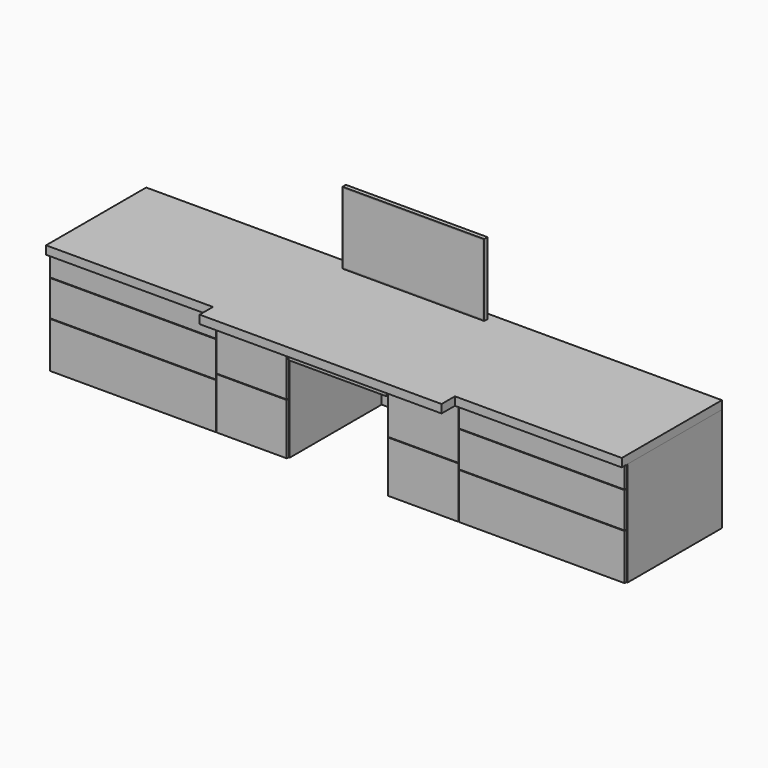
from build123d import *

# Parameters (mm, degrees)
F0_W       = 3505.2
F0_H       = 685.8
F1_DEPTH   = 381
F2_W       = 609.6
F2_H       = 635
F3_DEPTH   = 843.28
F5_W       = 596.9
F5_H       = 762
F6_DEPTH   = 19.05
F7_DEPTH   = 50.8
F8_W       = 1473.2
F8_H       = 101.6
F9_DEPTH   = 50.8
F7_FACE1_W = 1447.8
F7_FACE1_H = 635
F6_FACE_W  = 596.9
F6_FACE_H  = 19.05
F10_DEPTH  = 25.4
F11_W      = 1009.65
F11_H      = 127
F12_DEPTH  = 19.05
F11_H_2    = 215.9
F11_H_3    = 279.4
F11_W_2    = 428.625
F11_H_4    = 312.7375
F14_W      = 19.05
F14_H      = 635
F15_DEPTH  = 4173.22
F17_W      = 862.8043793142
F17_H      = 439.093708992
F17_W_2    = 850.1043793142
F17_H_2    = 426.393708992
F18_DEPTH  = 25.4
F19_DEPTH  = 25.4
F20_W      = 609.6
F20_H      = 635
F21_DEPTH  = 17.78


with BuildPart() as f1:
    # F0 (on Front) → F1 (new body, symmetric)
    with BuildSketch(Plane.XZ):
        with Locations((0, 469.9)):
            Rectangle(F0_W, F0_H)
    extrude(amount=F1_DEPTH, both=True)

    # F2 (on face) → F3 (cut)
    with BuildSketch(Plane.XZ.offset(381)):
        with Locations((0, 444.5)):
            Rectangle(F2_W, F2_H)
    extrude(amount=-F3_DEPTH, mode=Mode.SUBTRACT)

    # F7 (cut): a face of the model
    f7_faces = [f1.faces().sort_by_distance(p)[0] for p in [
        (0, 0, 812.8),
    ]]
    extrude(f7_faces, amount=-F7_DEPTH, mode=Mode.SUBTRACT)


with BuildPart() as f6:
    # F5 (on offset) → F6 (new body)
    with BuildSketch(Plane.XY.offset(660.4)):
        Rectangle(F5_W, F5_H)
    extrude(amount=F6_DEPTH)


with BuildPart() as f9:
    # F8 (on face) → F9 (new body)
    with BuildSketch(Plane.XY.offset(762)):
        Polygon((1752.6, 381), (-1752.6, 381), (-1752.6, -381), (-736.6, -381), (736.6, -381), (1752.6, -381), align=None)
        with Locations((0, -431.8)):
            Rectangle(F8_W, F8_H)
    extrude(amount=F9_DEPTH)


with BuildPart() as f10_tool:
    # F7_face1 (on face) + F6_face (on face) → F10 (new body)
    with BuildSketch(Plane(origin=(-1028.7, -381, 444.5), x_dir=(1, 0, 0), z_dir=(0, -1, 0))):
        Rectangle(F7_FACE1_W, F7_FACE1_H)
        with Locations((2057.4, 0)):
            Rectangle(F7_FACE1_W, F7_FACE1_H)
    with BuildSketch(Plane(origin=(0, -381, 669.925), x_dir=(1, 0, 0), z_dir=(0, -1, 0))):
        Rectangle(F6_FACE_W, F6_FACE_H)
    extrude(amount=-F10_DEPTH)


with BuildPart() as f1_1:
    add(f1.part)

    # F10: cut by f10_tool
    add(f10_tool.part, mode=Mode.SUBTRACT)


with BuildPart() as f6_1:
    add(f6.part)

    # F10: cut by f10_tool
    add(f10_tool.part, mode=Mode.SUBTRACT)


with BuildPart() as f12:
    # F11 (on face) → F12 (new body)
    with BuildSketch(Plane.XZ.offset(355.6)):
        with Locations((-1244.6, 695.325)):
            Rectangle(F11_W, F11_H)
    extrude(amount=-F12_DEPTH)


with BuildPart() as f12b:
    # F11 (on face) → F12, piece 2 (new body)
    with BuildSketch(Plane.XZ.offset(355.6)):
        with Locations((-1244.6, 520.7)):
            Rectangle(F11_W, F11_H_2)
    extrude(amount=-F12_DEPTH)


with BuildPart() as f12c:
    # F11 (on face) → F12, piece 3 (new body)
    with BuildSketch(Plane.XZ.offset(355.6)):
        with Locations((-1244.6, 269.875)):
            Rectangle(F11_W, F11_H_3)
    extrude(amount=-F12_DEPTH)


with BuildPart() as f12d:
    # F11 (on face) → F12, piece 4 (new body)
    with BuildSketch(Plane.XZ.offset(355.6)):
        with Locations((1244.6, 269.875)):
            Rectangle(F11_W, F11_H_3)
    extrude(amount=-F12_DEPTH)


with BuildPart() as f12e:
    # F11 (on face) → F12, piece 5 (new body)
    with BuildSketch(Plane.XZ.offset(355.6)):
        with Locations((1244.6, 695.325)):
            Rectangle(F11_W, F11_H)
    extrude(amount=-F12_DEPTH)


with BuildPart() as f12f:
    # F11 (on face) → F12, piece 6 (new body)
    with BuildSketch(Plane.XZ.offset(355.6)):
        with Locations((1244.6, 520.7)):
            Rectangle(F11_W, F11_H_2)
    extrude(amount=-F12_DEPTH)


with BuildPart() as f12g:
    # F11 (on face) → F12, piece 7 (new body)
    with BuildSketch(Plane.XZ.offset(355.6)):
        with Locations((-522.2875, 602.45625)):
            Rectangle(F11_W_2, F11_H_4)
    extrude(amount=-F12_DEPTH)


with BuildPart() as f12h:
    # F11 (on face) → F12, piece 8 (new body)
    with BuildSketch(Plane.XZ.offset(355.6)):
        with Locations((-522.2875, 286.54375)):
            Rectangle(F11_W_2, F11_H_4)
    extrude(amount=-F12_DEPTH)


with BuildPart() as f12i:
    # F11 (on face) → F12, piece 9 (new body)
    with BuildSketch(Plane.XZ.offset(355.6)):
        with Locations((522.2875, 602.45625)):
            Rectangle(F11_W_2, F11_H_4)
    extrude(amount=-F12_DEPTH)


with BuildPart() as f12j:
    # F11 (on face) → F12, piece 10 (new body)
    with BuildSketch(Plane.XZ.offset(355.6)):
        with Locations((522.2875, 286.54375)):
            Rectangle(F11_W_2, F11_H_4)
    extrude(amount=-F12_DEPTH)


with BuildPart() as f1_2:
    add(f1_1.part)

    # F13: cut F12j, F12, F12b, F12c, F12d, F12e, F12f, F12g, F12h, F12i
    add(f12j.part, mode=Mode.SUBTRACT)
    add(f12.part, mode=Mode.SUBTRACT)
    add(f12b.part, mode=Mode.SUBTRACT)
    add(f12c.part, mode=Mode.SUBTRACT)
    add(f12d.part, mode=Mode.SUBTRACT)
    add(f12e.part, mode=Mode.SUBTRACT)
    add(f12f.part, mode=Mode.SUBTRACT)
    add(f12g.part, mode=Mode.SUBTRACT)
    add(f12h.part, mode=Mode.SUBTRACT)
    add(f12i.part, mode=Mode.SUBTRACT)

    # F14 (on face) → F15 (cut)
    with BuildSketch(Plane(origin=(-1752.6, 0, 0), x_dir=(0, -1, 0), z_dir=(-1, 0, 0))):
        with Locations((346.075, 444.5)):
            Rectangle(F14_W, F14_H)
    extrude(amount=-F15_DEPTH, mode=Mode.SUBTRACT)


with BuildPart() as f18:
    # F17 (on offset) → F18 (new body)
    with BuildSketch(Plane(origin=(0, 223.52, 0), x_dir=(-1, 0, 0), z_dir=(0, 1, 0))):
        with Locations((0, 1091.0347700119)):
            Rectangle(F17_W, F17_H)
        with Locations((0, 1091.0347700119)):
            Rectangle(F17_W_2, F17_H_2, mode=Mode.SUBTRACT)
    extrude(amount=F18_DEPTH)


with BuildPart() as f19:
    # F17 (on offset) → F19 (new body)
    with BuildSketch(Plane(origin=(0, 223.52, 0), x_dir=(-1, 0, 0), z_dir=(0, 1, 0))):
        with Locations((0, 1091.0347700119)):
            Rectangle(F17_W_2, F17_H_2)
    extrude(amount=F19_DEPTH)


with BuildPart() as f21:
    # F20 (on face) → F21 (new body)
    with BuildSketch(Plane(origin=(0, 381, 0), x_dir=(-1, 0, 0), z_dir=(0, 1, 0))):
        with Locations((0, 444.5)):
            Rectangle(F20_W, F20_H)
    extrude(amount=-F21_DEPTH)


solid = Compound([f9.part, f6_1.part, f12.part, f12b.part, f12c.part, f12d.part, f12e.part, f12f.part, f12g.part, f12h.part, f12i.part, f12j.part, f1_2.part, f18.part, f19.part, f21.part])
